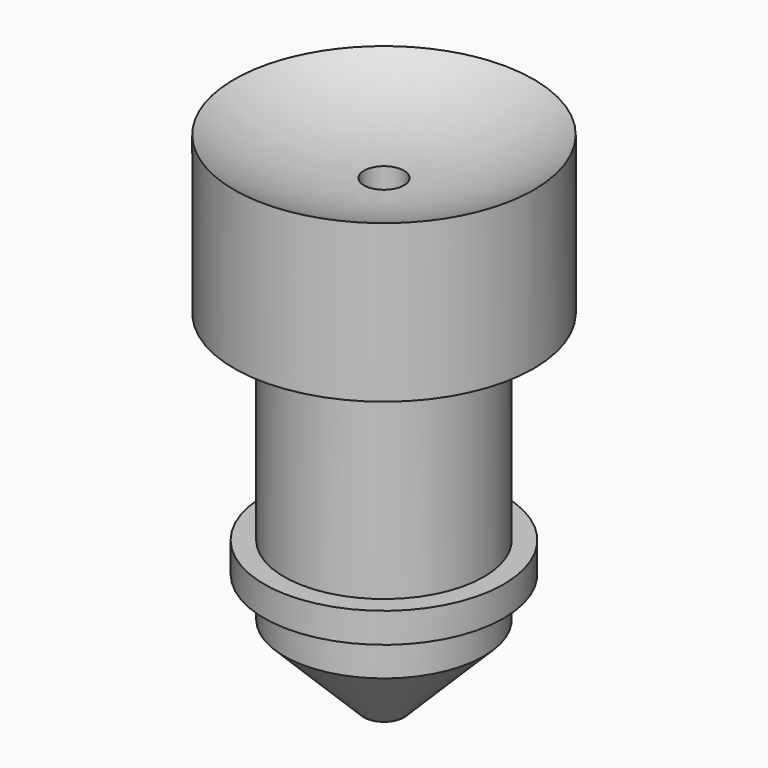
from build123d import *

# Parameters (mm, degrees)
F0_R      = 7.5
F1_DEPTH  = 10
F4_R      = 5
F5_DEPTH  = 18
F6_R      = 1
F7_DEPTH  = 25.8740546369
F10_R     = 6
F10_R_2   = 5
F11_DEPTH = 1.5


# Not quite as in the source:
# - a fillet or chamfer that OpenCascade refuses, or shapes differently, is made with other operations: its cross-section is extruded or revolved along the edge and cut away or added


with BuildPart() as f1:
    # F0 (on Top) → F1 (new body)
    with BuildSketch(Plane.XY):
        Circle(F0_R)
    extrude(amount=F1_DEPTH)

    # F2 (on Front) → F3 (revolve, cut)
    with BuildSketch(Plane.XZ):
        with BuildLine():
            Line((10, 10), (0, 10))
            Line((0, 10), (0, 6))
            ThreePointArc((0, 6), (5.4685094621, 6.8287263446), (10, 10))
        make_face()
    revolve(axis=Axis((0, 0, 8), (0, 0, -1)), mode=Mode.SUBTRACT)

    # F4 (on face) → F5 (join)
    with BuildSketch(Plane(origin=(0, 0, 0), x_dir=(1, 0, 0), z_dir=(0, 0, -1))):
        Circle(F4_R)
    extrude(amount=F5_DEPTH)

    # F6 (on face) → F7 (cut, through all)
    with BuildSketch(Plane(origin=(0, 0, -18), x_dir=(1, 0, 0), z_dir=(0, 0, -1))):
        Circle(F6_R)
    extrude(amount=-F7_DEPTH, mode=Mode.SUBTRACT)

    # F8: chamfer of 4.5 on 1 edges, made by hand

    # F8_s1 → F8_t2 (revolve, cut)
    with BuildSketch(Plane.XZ):
        Polygon((5, -13.5), (0.5, -18), (5, -18), align=None)
    revolve(axis=Axis((0, 0, -18), (0, 0, -1)), mode=Mode.SUBTRACT)

    # F10 (on offset) → F11 (join)
    with BuildSketch(Plane.XY.offset(-10)):
        Circle(F10_R)
        Circle(F10_R_2, mode=Mode.SUBTRACT)
    extrude(amount=-F11_DEPTH)


solid = f1.part
